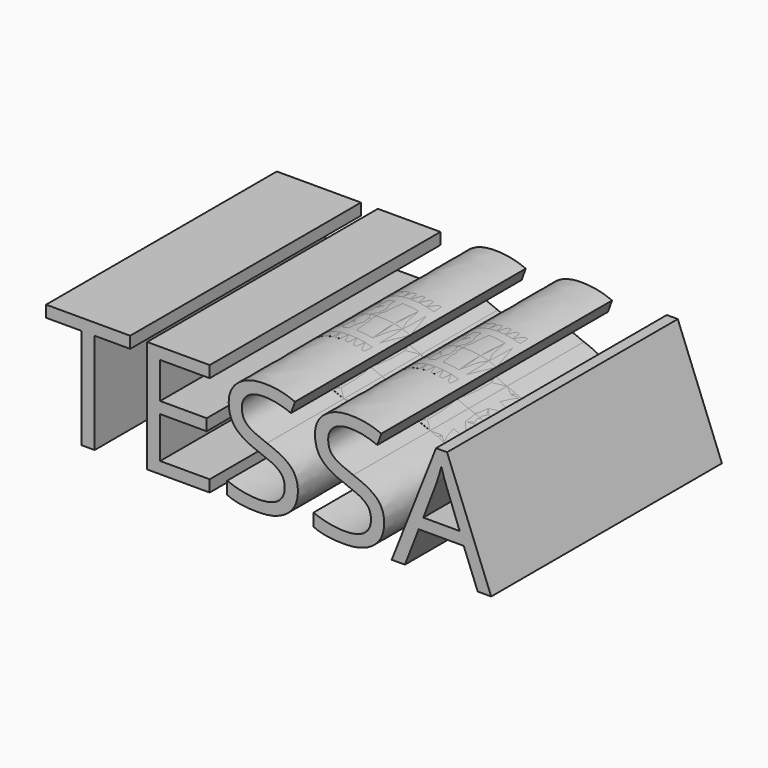
from build123d import *

# Parameters (mm, degrees)
F0_TEXT_SIZE = 41.534075628
F1_DEPTH     = 12.7
F2_DEPTH     = 38.1


# Not quite as in the source:
# - Text() gives the source's letters only with a copy of the font that has no kerning and outlines rounded to 1/6400 em; it was checked with that copy


with BuildPart() as f1:
    # F0 (on Front) → F1 (new body, symmetric)
    with BuildSketch(Plane.XZ):
        with Locations((0, -29.9045344522)):
            Text('TESSA', F0_TEXT_SIZE, font='Open Sans', text_align=(TextAlign.LEFT, TextAlign.BOTTOM))
    extrude(amount=F1_DEPTH, both=True)


with BuildPart() as f2:
    # F0 (on Front) → F2 (new body, symmetric)
    with BuildSketch(Plane.XZ):
        with Locations((0, -29.9045344522)):
            Text('TESSA', F0_TEXT_SIZE, font='Open Sans', text_align=(TextAlign.LEFT, TextAlign.BOTTOM))
    extrude(amount=F2_DEPTH, both=True)


solid = Compound([f1.part, f2.part])
